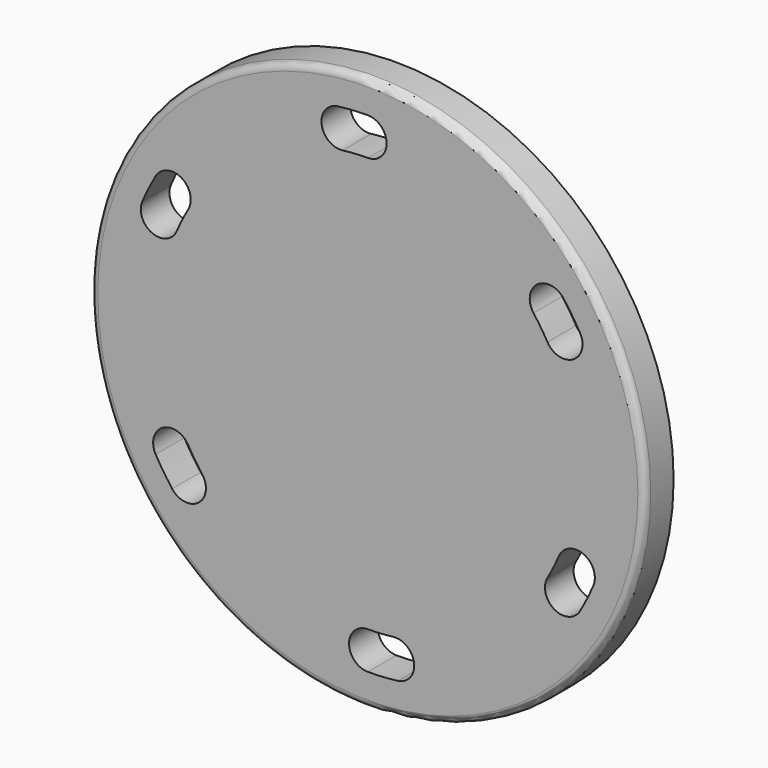
from build123d import *

# Parameters (mm, degrees)
F1_R            = 77.5
F2_DEPTH        = 10
F3_R            = 2
F4_DEPTH        = 10
F4_COPIES_COUNT = 6


# Not quite as in the source:
# - a pattern or mirror of a feature is missing from the dataset's text; its kind, count and spacing are read off the source's solid


with BuildPart() as f2:
    # F1 (on Front) → F2 (new body)
    with BuildSketch(Plane.XZ):
        Circle(F1_R)
    extrude(amount=-F2_DEPTH)

    # F3
    f3_edges = [f2.edges().sort_by_distance(p)[0] for p in [
        (-77.5, 0, 0),
    ]]
    fillet(f3_edges, radius=F3_R)

    # F0 (on Front) → F4 (cut, through all)
    with BuildSketch(Plane.XZ):
        with BuildLine():
            ThreePointArc((0, 68.5), (-4.1818249581, 68.3722336919), (-8.3480500233, 67.9894113874))
            ThreePointArc((-8.3480500233, 67.9894113874), (-12.9191032665, 62.1387300384), (-7.0684219175, 57.5676767952))
            ThreePointArc((-7.0684219175, 57.5676767952), (-3.540815293, 57.8918183085), (0, 58))
            ThreePointArc((0, 58), (5.25, 63.25), (0, 68.5))
        make_face()
    f4 = extrude(amount=-F4_DEPTH, mode=Mode.SUBTRACT)

    # F4_copies: F4 ×6 about axis
    f4_copies_axis = Axis((0, 0, 0), (0, 1, 0))
    for i in range(1, F4_COPIES_COUNT):
        add(f4.rotate(f4_copies_axis, i * 360 / F4_COPIES_COUNT), mode=Mode.SUBTRACT)


solid = f2.part
